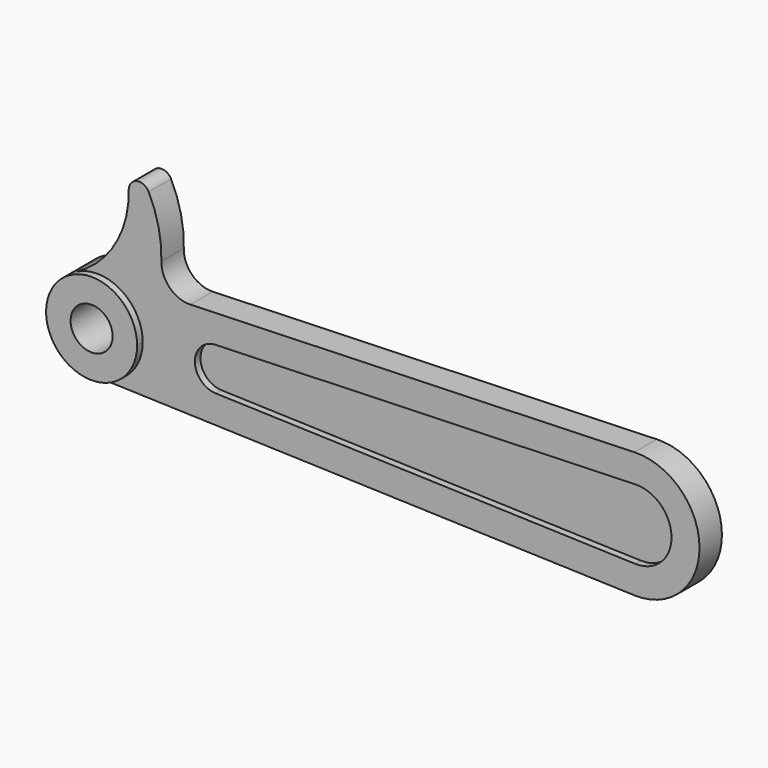
from build123d import *

# Parameters (mm, degrees)
F1_DEPTH = 2
F0_R     = 3
F2_DEPTH = 3
F3_DEPTH = 1


with BuildPart() as f1:
    # F0 (on Front) → F1 (new body, symmetric)
    with BuildSketch(Plane.XZ):
        with BuildLine():
            ThreePointArc((-3.011066, 5.760511), (3.367348, 5.559763), (6.5, 0))
            ThreePointArc((6.5, 0), (4.520965, -4.670212), (-0.211039, -6.496573))
            Line((-0.211039, -6.496573), (76.707792, -8.995255))
            ThreePointArc((76.707792, -8.995255), (86, 0), (76.707792, 8.995255))
            Line((76.707792, 8.995255), (13.292901, 6.935244))
            ThreePointArc((13.292901, 6.935244), (10.342359, 8.096974), (9.164489, 11.041109))
            ThreePointArc((9.164489, 11.041109), (8.758012, 15.222971), (7.338321, 19.177419))
            ThreePointArc((7.338321, 19.177419), (5.636159, 19.955204), (4.500345, 18.467848))
            ThreePointArc((4.500345, 18.467848), (2.555482, 11.043776), (-3.011066, 5.760511))
        make_face()
        with BuildLine():
            ThreePointArc((76.837662, 4.997364), (82, 0), (76.837662, -4.997364))
            Line((76.837662, -4.997364), (16.900911, -3.050339))
            ThreePointArc((16.900911, -3.050339), (13.948052, 0), (16.900911, 3.050339))
            Line((16.900911, 3.050339), (76.837662, 4.997364))
        make_face(mode=Mode.SUBTRACT)
    extrude(amount=F1_DEPTH, both=True)

    # F0 (on Front) → F2 (join, symmetric)
    with BuildSketch(Plane.XZ):
        with BuildLine():
            ThreePointArc((-0.211039, -6.496573), (4.520965, -4.670212), (6.5, 0))
            ThreePointArc((6.5, 0), (3.367348, 5.559763), (-3.011066, 5.760511))
            ThreePointArc((-3.011066, 5.760511), (-6.336759, -1.447579), (-0.211039, -6.496573))
        make_face()
        Circle(F0_R, mode=Mode.SUBTRACT)
    extrude(amount=F2_DEPTH, both=True)

    # F0 (on Front) → F3 (join, symmetric)
    with BuildSketch(Plane.XZ):
        with BuildLine():
            Line((16.900911, -3.050339), (76.837662, -4.997364))
            ThreePointArc((76.837662, -4.997364), (82, 0), (76.837662, 4.997364))
            Line((76.837662, 4.997364), (16.900911, 3.050339))
            ThreePointArc((16.900911, 3.050339), (13.948052, 0), (16.900911, -3.050339))
        make_face()
    extrude(amount=F3_DEPTH, both=True)


solid = f1.part
